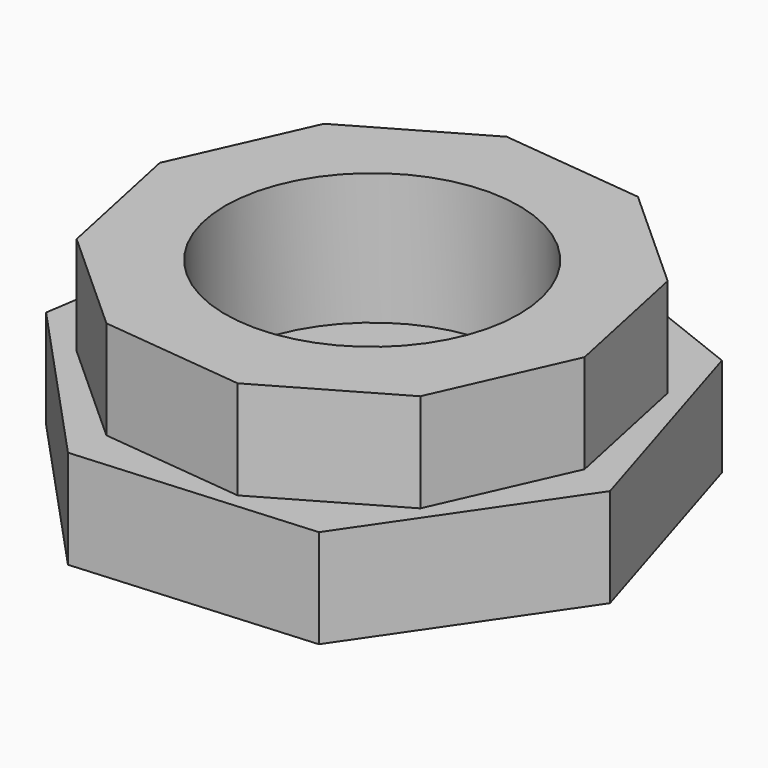
from build123d import *

# Parameters (mm, degrees)
F1_DEPTH     = 15.24
F3_DEPTH     = 15.24
F4_R         = 22.684578283
F5_DEPTH     = 20.32
F6_TEXT_SIZE = 13.3253183234
F7_DEPTH     = 2.54


# Not quite as in the source:
# - Text() gives the source's letters only with a copy of the font that has no kerning and outlines rounded to 1/6400 em; it was checked with that copy


with BuildPart() as f1:
    # F0 (on Top) → F1 (new body)
    with BuildSketch(Plane.XY):
        Polygon((-3.1041826599, 42.1737228174), (-34.9081704631, 23.8679383523), (-40.4255939107, -12.4108905094), (-15.5017206117, -39.3440656814), (21.0952644854, -36.6503569227), (41.80708516, -6.3581818701), (31.037318, 28.7218338139), align=None)
    extrude(amount=F1_DEPTH)

    # F2 (on face) → F3 (join)
    with BuildSketch(Plane.XY.offset(15.24)):
        Polygon((-7.4493524867, 35.2766805298), (-26.761765324, 24.1608145229), (-35.8520934066, 3.8163385642), (-31.2481403756, -17.9858490135), (-14.7084598064, -32.9180535845), (7.4493524867, -35.2766805298), (26.761765324, -24.1608145229), (35.8520934066, -3.8163385642), (31.2481403756, 17.9858490135), (14.7084598064, 32.9180535845), align=None)
    extrude(amount=F3_DEPTH)

    # F4 (on face) → F5 (cut)
    with BuildSketch(Plane.XY.offset(30.48)):
        Circle(F4_R)
    extrude(amount=-F5_DEPTH, mode=Mode.SUBTRACT)

    # F6 (on face) → F7 (cut)
    with BuildSketch(Plane.XY.offset(10.16)):
        with Locations((-19.3461598342, -5.0034499233)):
            Text('K.B.R.', F6_TEXT_SIZE, font='Open Sans', font_style=FontStyle.BOLD, text_align=(TextAlign.LEFT, TextAlign.BOTTOM))
    extrude(amount=-F7_DEPTH, mode=Mode.SUBTRACT)


solid = f1.part
